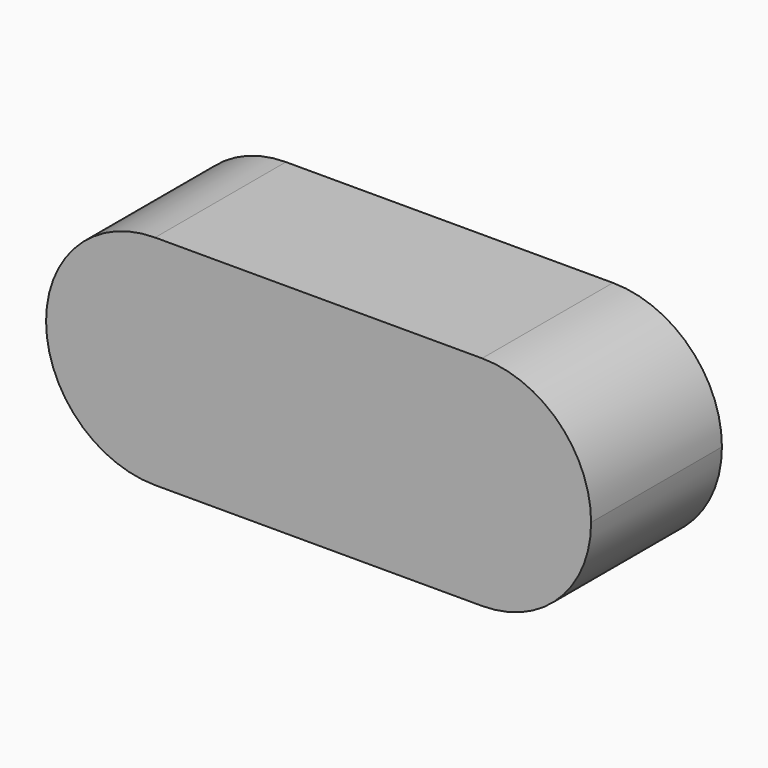
from build123d import *

# Parameters (mm, degrees)
F0_W     = 127
F0_H     = 50.8
F1_DEPTH = 38.1
F2_R     = 25.39999
F3_R     = 12.2082879552
F3_R_2   = 12.7
F4_DEPTH = 19.05


# Not quite as in the source:
# - a fillet or chamfer is up to 0.001 mm smaller than in the source, because OpenCascade refuses the exact size


with BuildPart() as f1:
    # F0 (on Front) → F1 (new body)
    with BuildSketch(Plane.XZ):
        Rectangle(F0_W, F0_H)
    extrude(amount=F1_DEPTH)

    # F2 (radius 25.4 in the source; OpenCascade refuses exactly that, so slightly less here)
    f2_edges = [f1.edges().sort_by_distance(p)[0] for p in [
        (63.5, -19.05, 25.4),
        (63.5, -19.05, -25.4),
        (-63.5, -19.05, 25.4),
        (-63.5, -19.05, -25.4),
    ]]
    fillet(f2_edges, radius=F2_R)

    # F3 (on face) → F4 (cut)
    with BuildSketch(Plane(origin=(0, 0, 0), x_dir=(-1, 0, 0), z_dir=(0, 1, 0))):
        with Locations((47.625, 0)):
            Circle(F3_R)
        with Locations((-47.625, 0)):
            Circle(F3_R_2)
    extrude(amount=-F4_DEPTH, mode=Mode.SUBTRACT)


solid = f1.part
